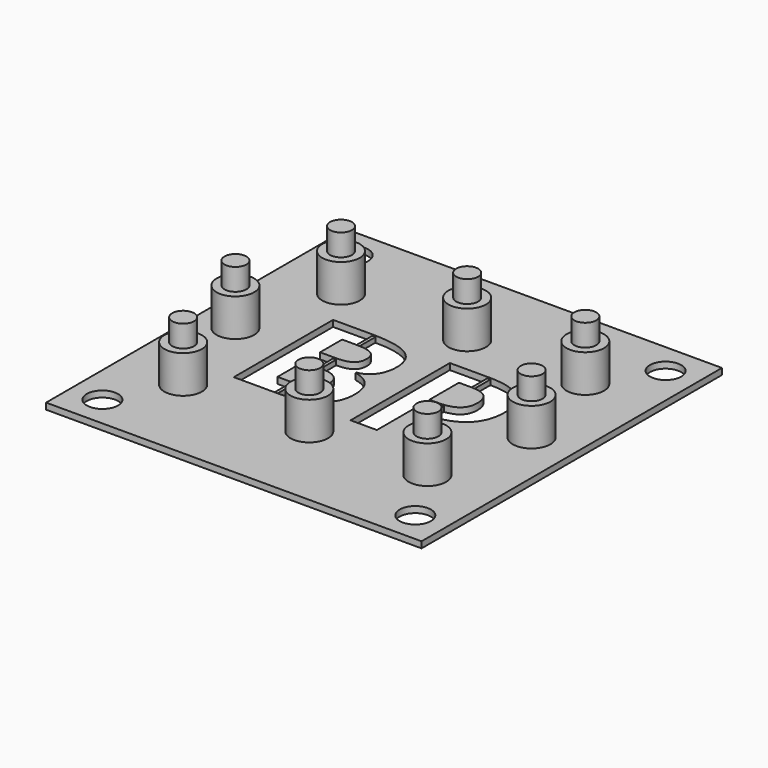
from build123d import *

# Parameters (mm, degrees)
F0_W         = 120
F0_H         = 120
F1_DEPTH     = 2
F2_R         = 5
F2_TEXT_SIZE = 55.5555555556
F3_DEPTH     = 25
F4_R         = 6
F6_DEPTH     = 12
F5_R         = 3.5
F7_DEPTH     = 19
F8_W         = 1
F8_H         = 70
F9_DEPTH     = 1.6


# Not quite as in the source:
# - Text() gives the source's letters only with a copy of the font that has no kerning and outlines rounded to 1/6400 em; it was checked with that copy


with BuildPart() as f1:
    # F0 (on Top) → F1 (new body)
    with BuildSketch(Plane.XY):
        with Locations((-1, 0)):
            Rectangle(F0_W, F0_H)
    extrude(amount=F1_DEPTH)

    # F2 (on face) → F3 (cut)
    with BuildSketch(Plane.XY.offset(2)):
        with Locations((-51, -50)):
            Circle(F2_R)
        with Locations((-51, 50)):
            Circle(F2_R)
        with Locations((49, 50)):
            Circle(F2_R)
        with Locations((49, -50)):
            Circle(F2_R)
        with Locations((-38, -20)):
            Text('BP', F2_TEXT_SIZE, font='Open Sans', font_style=FontStyle.BOLD, text_align=(TextAlign.LEFT, TextAlign.BOTTOM))
    extrude(amount=-F3_DEPTH, mode=Mode.SUBTRACT)

    # F4 (on face) → F6 (join)
    with BuildSketch(Plane.XY.offset(2)):
        with Locations((-40.3221660001, -31.0879173718)):
            Circle(F4_R)
        with Locations((0, -31.0879173718)):
            Circle(F4_R)
        with Locations((37.7502330675, -31.087918207)):
            Circle(F4_R)
        with Locations((-40.3221659362, 31.9815091789)):
            Circle(F4_R)
        with Locations((6.39e-08, 31.9815091789)):
            Circle(F4_R)
        with Locations((37.7502331315, 31.9815083436)):
            Circle(F4_R)
        with Locations((-49.2942109704, 1)):
            Circle(F4_R)
        with Locations((45.3722976158, 1)):
            Circle(F4_R)
    extrude(amount=F6_DEPTH)

    # F5 (on face) → F7 (join)
    with BuildSketch(Plane.XY.offset(2)):
        with Locations((-40.3221660001, -31.0879173718)):
            Circle(F5_R)
        with Locations((0, -31.0879173718)):
            Circle(F5_R)
        with Locations((37.7637186823, -31.087918207)):
            Circle(F5_R)
        with Locations((-40.3221659362, 31.9815091789)):
            Circle(F5_R)
        with Locations((6.39e-08, 31.9815091789)):
            Circle(F5_R)
        with Locations((37.7502331315, 31.9815083436)):
            Circle(F5_R)
        with Locations((-49.2807253556, 1)):
            Circle(F5_R)
        with Locations((45.3722976158, 1)):
            Circle(F5_R)
    extrude(amount=F7_DEPTH)


with BuildPart() as f9:
    # F8 (on Top) → F9 (new body)
    with BuildSketch(Plane.XY):
        with Locations((-19.9435390532, 5)):
            Rectangle(F8_W, F8_H)
    extrude(amount=F9_DEPTH)


with BuildPart() as f9b:
    # F8 (on Top) → F9, piece 2 (new body)
    with BuildSketch(Plane.XY):
        with Locations((16.8137745112, 4.3833943456)):
            Rectangle(F8_W, F8_H)
    extrude(amount=F9_DEPTH)


solid = Compound([f1.part, f9.part, f9b.part])
